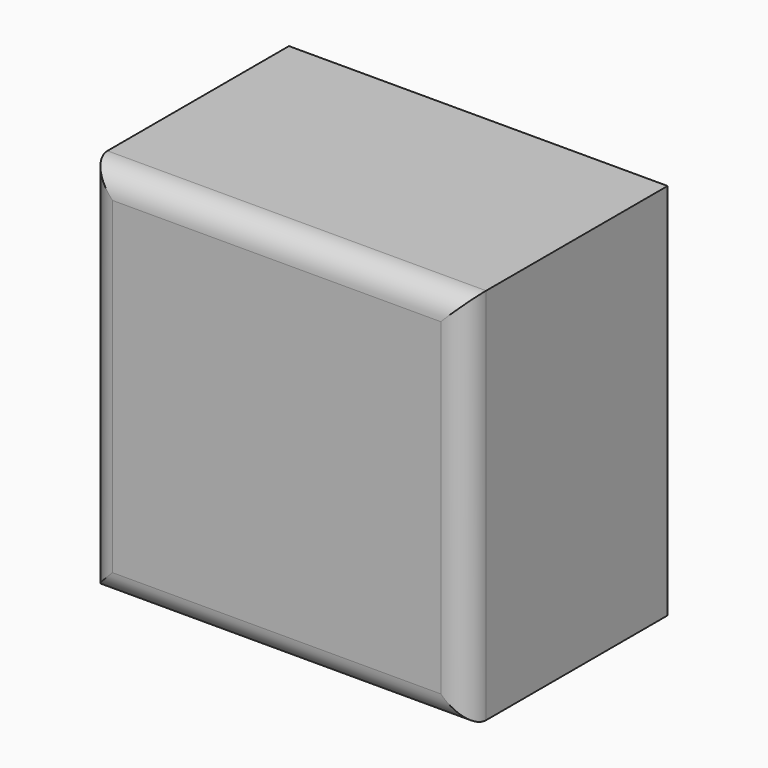
from build123d import *

# Parameters (mm, degrees)
F0_W     = 76.3154625893
F0_H     = 76.2000009418
F1_DEPTH = 25.4
F2_R     = 5.08


with BuildPart() as f1:
    # F0 (on Front) → F1 (new body, symmetric)
    with BuildSketch(Plane.XZ):
        with Locations((38.1577312946, 38.1000004709)):
            Rectangle(F0_W, F0_H)
    extrude(amount=F1_DEPTH, both=True)

    # F2
    f2_edges = [f1.edges().sort_by_distance(p)[0] for p in [
        (38.157731, -25.4, 76.200001),
        (76.315463, -25.4, 38.1),
        (38.157731, -25.4, 0),
        (0, -25.4, 38.1),
    ]]
    fillet(f2_edges, radius=F2_R)


solid = f1.part
